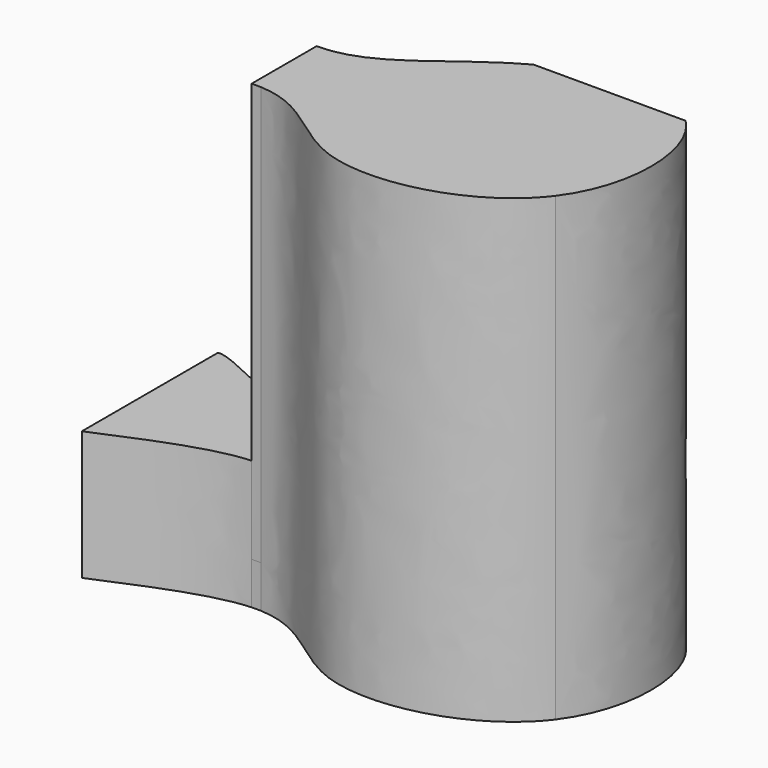
from build123d import *

# Parameters (mm, degrees)
F1_DEPTH = 3.9
F2_DEPTH = 11.9
F3_DEPTH = 42.5


with BuildPart() as f1:
    # F0 (on Top) → F1 (new body)
    with BuildSketch(Plane.XY):
        with BuildLine():
            Line((15.2110805884, -1.0073357602), (1.2110805884, -1.0073357602))
            Line((1.2110805884, -1.0073357602), (1.2110805884, -8.5073357602))
            add(Edge.make_bspline(
                [(15.2110805884, -1.0073357602), (10.1056651112, -3.7045784545), (6.4222975956, -8.6121569817), (1.2110805884, -8.5073357602)],
                knots=[0.5948688465, 0.5948688465, 0.5948688465, 0.5948688465, 0.7145243028, 0.7145243028, 0.7145243028, 0.7145243028], degree=3))
        make_face()
        with BuildLine():
            Line((29.2110805884, -1.0073357602), (15.2110805884, -1.0073357602))
            add(Edge.make_bspline(
                [(15.2110805884, -1.0073357602), (10.1056651112, -3.7045784545), (6.4222975956, -8.6121569817), (1.2110805884, -8.5073357602)],
                knots=[0.5948688465, 0.5948688465, 0.5948688465, 0.5948688465, 0.7145243028, 0.7145243028, 0.7145243028, 0.7145243028], degree=3))
            Line((1.2110805884, -8.5073357602), (1.2110805884, -16.0073357602))
            add(Edge.make_bspline(
                [(1.2110805884, -16.0073357602), (1.5073310932, -15.9933259222), (1.7934505794, -15.9937789675), (2.0704529167, -16.0073357602)],
                knots=[0.1348057981, 0.1348057981, 0.1348057981, 0.1348057981, 0.1410104438, 0.1410104438, 0.1410104438, 0.1410104438], degree=3))
            Line((2.0704529167, -16.0073357602), (29.2110805884, -16.0073357602))
            Line((29.2110805884, -16.0073357602), (29.2110805884, -1.0073357602))
        make_face()
    extrude(amount=F1_DEPTH)

    # F0 (on Top) → F2 (join)
    with BuildSketch(Plane.XY):
        with BuildLine():
            Line((1.2110805884, -16.0073357602), (1.2110805884, -8.5073357602))
            add(Edge.make_bspline(
                [(1.2110805884, -8.5073357602), (-3.5186716625, -8.4121989798), (-9.506998743, -4.1880690008), (-11.1998226494, -4.3673282489)],
                knots=[0.7145243028, 0.7145243028, 0.7145243028, 0.7145243028, 0.823124782, 0.823124782, 0.823124782, 0.823124782], degree=3))
            Line((-11.1998226499, -4.367328249), (-11.1998226499, -20.0583143803))
            add(Edge.make_bspline(
                [(-11.1998226499, -20.0583143803), (-7.1868911838, -18.3499221531), (-2.2831850449, -16.1725813711), (1.2110805884, -16.0073357602)],
                knots=[0.0616221929, 0.0616221929, 0.0616221929, 0.0616221929, 0.1348057981, 0.1348057981, 0.1348057981, 0.1348057981], degree=3))
        make_face()
    extrude(amount=F2_DEPTH)

    # F0 (on Top) → F3 (join)
    with BuildSketch(Plane.XY):
        with BuildLine():
            Line((29.2110805884, -1.0073357602), (15.2110805884, -1.0073357602))
            add(Edge.make_bspline(
                [(15.2110805884, -1.0073357602), (10.1056651112, -3.7045784545), (6.4222975956, -8.6121569817), (1.2110805884, -8.5073357602)],
                knots=[0.5948688465, 0.5948688465, 0.5948688465, 0.5948688465, 0.7145243028, 0.7145243028, 0.7145243028, 0.7145243028], degree=3))
            Line((1.2110805884, -8.5073357602), (1.2110805884, -16.0073357602))
            add(Edge.make_bspline(
                [(1.2110805884, -16.0073357602), (1.5073310932, -15.9933259222), (1.7934505794, -15.9937789675), (2.0704529167, -16.0073357602)],
                knots=[0.1348057981, 0.1348057981, 0.1348057981, 0.1348057981, 0.1410104438, 0.1410104438, 0.1410104438, 0.1410104438], degree=3))
            Line((2.0704529167, -16.0073357602), (29.2110805884, -16.0073357602))
            Line((29.2110805884, -16.0073357602), (29.2110805884, -1.0073357602))
        make_face()
        with BuildLine():
            add(Edge.make_bspline(
                [(29.2110805884, -16.0073357602), (32.6593398461, -11.4234913165), (32.4818190242, -4.2330775311), (29.2110805884, -1.0073357602)],
                knots=[0.3662436292, 0.3662436292, 0.3662436292, 0.3662436292, 0.4825277311, 0.4825277311, 0.4825277311, 0.4825277311], degree=3))
            Line((29.2110805884, -1.0073357602), (29.2110805884, -16.0073357602))
        make_face()
        with BuildLine():
            add(Edge.make_bspline(
                [(2.0704529167, -16.0073357602), (6.535385921, -16.225854391), (11.2561235238, -24.3852753557), (25.4977786279, -20.9435071114), (29.2110805884, -16.0073357602)],
                knots=[0.1410104438, 0.1410104438, 0.1410104438, 0.1410104438, 0.2410216109, 0.3662436292, 0.3662436292, 0.3662436292, 0.3662436292], degree=3))
            Line((29.2110805884, -16.0073357602), (2.0704529167, -16.0073357602))
        make_face()
    extrude(amount=F3_DEPTH)


solid = f1.part
